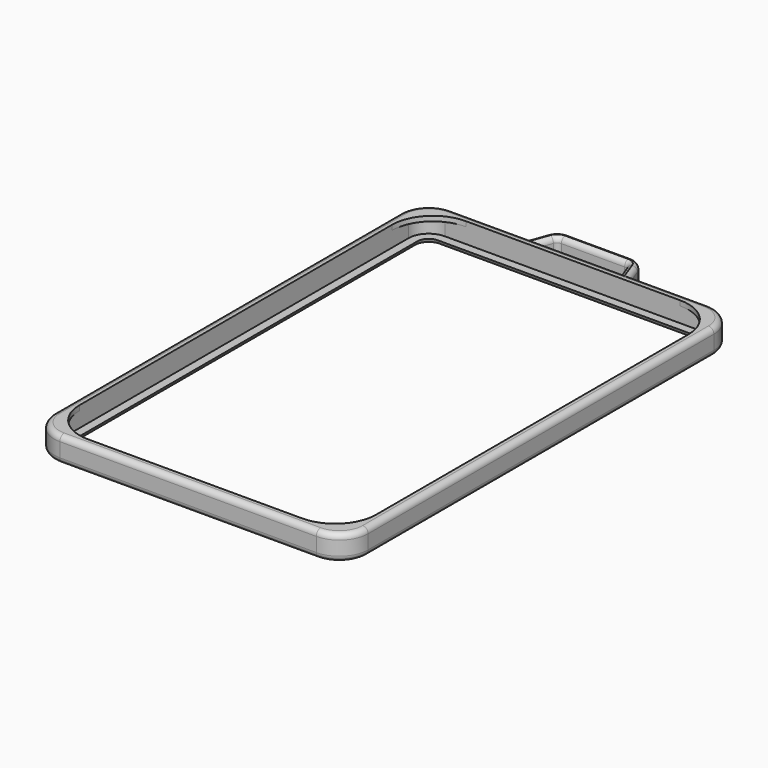
from build123d import *

# Parameters (mm, degrees)
F1_DEPTH      = 2.8
F3_DEPTH      = 0.9
F5_DEPTH      = 0.9
F7_DEPTH      = 3.7
F7_DEPTH_BACK = 0.9
F8_T1_DEPTH   = 79.2801919127
F8_T3_DEPTH   = 11.5995849236
F8_T5_DEPTH   = 47.0301919127
F8_T10_DEPTH  = 4.9923257792
F8_T15_DEPTH  = 20.1838214056
F8_T20_DEPTH  = 20.1838214056
F8_T26_DEPTH  = 20.1838214056
F8_T31_DEPTH  = 20.1838214056
F8_T36_DEPTH  = 20.1838214056
F8_T42_DEPTH  = 20.1838214056
F8_T45_ANGLE  = 90
F8_T47_ANGLE  = 90
F8_T49_ANGLE  = 90
F8_T51_ANGLE  = 90
F8_T53_ANGLE  = 90
F8_T57_DEPTH  = 16.7205008176
F8_T62_DEPTH  = 16.7205008176
F8_T67_DEPTH  = 16.7205008176
F8_T72_DEPTH  = 16.7205008176
F8_T75_ANGLE  = 90
F8_T77_ANGLE  = 90
F8_T81_DEPTH  = 16.7205008176
F8_T86_DEPTH  = 16.7205008176
F8_T91_DEPTH  = 16.7205008176
F8_T96_DEPTH  = 16.7205008176
F8_T99_ANGLE  = 90
F8_T101_ANGLE = 90
F8_T103_ANGLE = 90
F8_T105_ANGLE = 90
F8_T107_ANGLE = 90
F8_T109_ANGLE = 70
F8_T111_ANGLE = 70
F8_T115_DEPTH = 4.9923257792
F8_T120_DEPTH = 4.9923257792
F8_T123_ANGLE = 70
F8_T125_ANGLE = 70
F8_T129_DEPTH = 5.574678154
F8_T134_DEPTH = 5.574678154
F8_T137_ANGLE = 70
F8_T139_ANGLE = 70
F8_T143_DEPTH = 5.574678154
F8_T148_DEPTH = 5.574678154
F8_T151_ANGLE = 70
F8_T153_ANGLE = 70
F8_T157_DEPTH = 4.9923257792
F8_T163_DEPTH = 20.1838214056
F8_T168_DEPTH = 4.9923257792
F8_T175_DEPTH = 20.1838214056
F8_T180_DEPTH = 4.9923257792
F8_T187_DEPTH = 20.1838214056
F8_T192_DEPTH = 4.9923257792
F8_T199_DEPTH = 20.1838214056
F8_T204_DEPTH = 4.9923257792
F8_T211_DEPTH = 16.7205008176
F8_T216_DEPTH = 5.574678154
F8_T223_DEPTH = 5.574678154
F8_T227_DEPTH = 16.7205008176
F8_T235_DEPTH = 16.7205008176
F8_T240_DEPTH = 5.574678154
F8_T247_DEPTH = 5.574678154
F8_T251_DEPTH = 16.7205008176


# Not quite as in the source:
# - a fillet or chamfer that OpenCascade refuses, or shapes differently, is made with other operations: its cross-section is extruded or revolved along the edge and cut away or added


with BuildPart() as f1:
    # F0 (on Top) → F1 (new body)
    with BuildSketch(Plane.XY):
        with BuildLine():
            Line((-28.8, 39.6400959564), (-28.8, -39.6400959564))
            ThreePointArc((-28.8, -39.6400959564), (-27.2520874435, -43.3770874435), (-23.5150959564, -44.925))
            Line((-23.5150959564, -44.925), (23.5150959564, -44.925))
            ThreePointArc((23.5150959564, -44.925), (27.2520874435, -43.3770874435), (28.8, -39.6400959564))
            Line((28.8, -39.6400959564), (28.8, 39.6400959564))
            ThreePointArc((28.8, 39.6400959564), (27.2520874435, 43.3770874435), (23.5150959564, 44.925))
            Line((23.5150959564, 44.925), (-23.5150959564, 44.925))
            ThreePointArc((-23.5150959564, 44.925), (-27.2520874435, 43.3770874435), (-28.8, 39.6400959564))
        make_face()
        with BuildLine():
            ThreePointArc((-23.5150959564, -43.325), (-26.1207165936, -42.2457165936), (-27.2, -39.6400959564))
            Line((-27.2, -39.6400959564), (-27.2, 39.6400959564))
            ThreePointArc((-27.2, 39.6400959564), (-26.1207165936, 42.2457165936), (-23.5150959564, 43.325))
            Line((-23.5150959564, 43.325), (23.5150959564, 43.325))
            ThreePointArc((23.5150959564, 43.325), (26.1207165936, 42.2457165936), (27.2, 39.6400959564))
            Line((27.2, 39.6400959564), (27.2, -39.6400959564))
            ThreePointArc((27.2, -39.6400959564), (26.1207165936, -42.2457165936), (23.5150959564, -43.325))
            Line((23.5150959564, -43.325), (-23.5150959564, -43.325))
        make_face(mode=Mode.SUBTRACT)
    extrude(amount=F1_DEPTH)

    # F2 (on face) → F3 (join)
    with BuildSketch(Plane(origin=(0, 0, 0), x_dir=(1, 0, 0), z_dir=(0, 0, -1))):
        with BuildLine():
            Line((28.8, -39.6400959564), (28.8, 39.6400959564))
            ThreePointArc((28.8, 39.6400959564), (27.2520874435, 43.3770874435), (23.5150959564, 44.925))
            Line((23.5150959564, 44.925), (-23.5150959564, 44.925))
            ThreePointArc((-23.5150959564, 44.925), (-27.2520874435, 43.3770874435), (-28.8, 39.6400959564))
            Line((-28.8, 39.6400959564), (-28.8, -39.6400959564))
            ThreePointArc((-28.8, -39.6400959564), (-27.2520874435, -43.3770874435), (-23.5150959564, -44.925))
            Line((-23.5150959564, -44.925), (23.5150959564, -44.925))
            ThreePointArc((23.5150959564, -44.925), (27.2520874435, -43.3770874435), (28.8, -39.6400959564))
        make_face()
        with BuildLine():
            Line((-27.2, -39.6400959564), (-27.2, 39.6400959564))
            ThreePointArc((-27.2, 39.6400959564), (-26.1207165936, 42.2457165936), (-23.5150959564, 43.325))
            Line((-23.5150959564, 43.325), (23.5150959564, 43.325))
            ThreePointArc((23.5150959564, 43.325), (26.1207165936, 42.2457165936), (27.2, 39.6400959564))
            Line((27.2, 39.6400959564), (27.2, -39.6400959564))
            ThreePointArc((27.2, -39.6400959564), (26.1207165936, -42.2457165936), (23.5150959564, -43.325))
            Line((23.5150959564, -43.325), (-23.5150959564, -43.325))
            ThreePointArc((-23.5150959564, -43.325), (-26.1207165936, -42.2457165936), (-27.2, -39.6400959564))
        make_face(mode=Mode.SUBTRACT)
        with BuildLine():
            ThreePointArc((-23.5150959564, 43.325), (-26.1207165936, 42.2457165936), (-27.2, 39.6400959564))
            Line((-27.2, 39.6400959564), (-27.2, -39.6400959564))
            ThreePointArc((-27.2, -39.6400959564), (-26.1207165936, -42.2457165936), (-23.5150959564, -43.325))
            Line((-23.5150959564, -43.325), (23.5150959564, -43.325))
            ThreePointArc((23.5150959564, -43.325), (26.1207165936, -42.2457165936), (27.2, -39.6400959564))
            Line((27.2, -39.6400959564), (27.2, 39.6400959564))
            ThreePointArc((27.2, 39.6400959564), (26.1207165936, 42.2457165936), (23.5150959564, 43.325))
            Line((23.5150959564, 43.325), (-23.5150959564, 43.325))
        make_face()
        with BuildLine():
            Line((-25.6, -39.6400959564), (-25.6, 39.6400959564))
            ThreePointArc((-25.6, 39.6400959564), (-24.9893457437, 41.1143457437), (-23.5150959564, 41.725))
            Line((-23.5150959564, 41.725), (23.5150959564, 41.725))
            ThreePointArc((23.5150959564, 41.725), (24.9893457437, 41.1143457437), (25.6, 39.6400959564))
            Line((25.6, 39.6400959564), (25.6, -39.6400959564))
            ThreePointArc((25.6, -39.6400959564), (24.9893457437, -41.1143457437), (23.5150959564, -41.725))
            Line((23.5150959564, -41.725), (-23.5150959564, -41.725))
            ThreePointArc((-23.5150959564, -41.725), (-24.9893457437, -41.1143457437), (-25.6, -39.6400959564))
        make_face(mode=Mode.SUBTRACT)
    extrude(amount=F3_DEPTH)

    # F4 (on face) → F5 (join)
    with BuildSketch(Plane.XY.offset(2.8)):
        with BuildLine():
            Line((-23.5150959564, -44.925), (23.5150959564, -44.925))
            ThreePointArc((23.5150959564, -44.925), (27.2520874435, -43.3770874435), (28.8, -39.6400959564))
            Line((28.8, -39.6400959564), (28.8, 39.6400959564))
            ThreePointArc((28.8, 39.6400959564), (27.2520874435, 43.3770874435), (23.5150959564, 44.925))
            Line((23.5150959564, 44.925), (-23.5150959564, 44.925))
            ThreePointArc((-23.5150959564, 44.925), (-27.2520874435, 43.3770874435), (-28.8, 39.6400959564))
            Line((-28.8, 39.6400959564), (-28.8, -39.6400959564))
            ThreePointArc((-28.8, -39.6400959564), (-27.2520874435, -43.3770874435), (-23.5150959564, -44.925))
        make_face()
        with BuildLine():
            Line((19.6523542566, 43.325), (23.5150959564, 43.325))
            ThreePointArc((23.5150959564, 43.325), (26.1207165936, 42.2457165936), (27.2, 39.6400959564))
            Line((27.2, 39.6400959564), (27.2, 35.7773542566))
            Line((27.2, 35.7773542566), (27.2, -35.7773542566))
            Line((27.2, -35.7773542566), (27.2, -39.6400959564))
            ThreePointArc((27.2, -39.6400959564), (26.1207165936, -42.2457165936), (23.5150959564, -43.325))
            Line((23.5150959564, -43.325), (19.6523542566, -43.325))
            Line((19.6523542566, -43.325), (-19.6523542566, -43.325))
            Line((-19.6523542566, -43.325), (-23.5150959564, -43.325))
            ThreePointArc((-23.5150959564, -43.325), (-26.1207165936, -42.2457165936), (-27.2, -39.6400959564))
            Line((-27.2, -39.6400959564), (-27.2, -35.7773542566))
            Line((-27.2, -35.7773542566), (-27.2, 35.7773542566))
            Line((-27.2, 35.7773542566), (-27.2, 39.6400959564))
            ThreePointArc((-27.2, 39.6400959564), (-26.1207165936, 42.2457165936), (-23.5150959564, 43.325))
            Line((-23.5150959564, 43.325), (-19.6523542566, 43.325))
            Line((-19.6523542566, 43.325), (19.6523542566, 43.325))
        make_face(mode=Mode.SUBTRACT)
        with BuildLine():
            ThreePointArc((-27.2, 35.7773542566), (-24.9893457437, 41.1143457437), (-19.6523542566, 43.325))
            Line((-19.6523542566, 43.325), (-23.5150959564, 43.325))
            ThreePointArc((-23.5150959564, 43.325), (-26.1207165936, 42.2457165936), (-27.2, 39.6400959564))
            Line((-27.2, 39.6400959564), (-27.2, 35.7773542566))
        make_face()
        with BuildLine():
            ThreePointArc((27.2, 39.6400959564), (26.1207165936, 42.2457165936), (23.5150959564, 43.325))
            Line((23.5150959564, 43.325), (19.6523542566, 43.325))
            ThreePointArc((19.6523542566, 43.325), (24.9893457437, 41.1143457437), (27.2, 35.7773542566))
            Line((27.2, 35.7773542566), (27.2, 39.6400959564))
        make_face()
        with BuildLine():
            Line((27.2, -39.6400959564), (27.2, -35.7773542566))
            ThreePointArc((27.2, -35.7773542566), (24.9893457437, -41.1143457437), (19.6523542566, -43.325))
            Line((19.6523542566, -43.325), (23.5150959564, -43.325))
            ThreePointArc((23.5150959564, -43.325), (26.1207165936, -42.2457165936), (27.2, -39.6400959564))
        make_face()
        with BuildLine():
            ThreePointArc((-19.6523542566, -43.325), (-24.9893457437, -41.1143457437), (-27.2, -35.7773542566))
            Line((-27.2, -35.7773542566), (-27.2, -39.6400959564))
            ThreePointArc((-27.2, -39.6400959564), (-26.1207165936, -42.2457165936), (-23.5150959564, -43.325))
            Line((-23.5150959564, -43.325), (-19.6523542566, -43.325))
        make_face()
    extrude(amount=F5_DEPTH)

    # F6 (on Top) → F7 (join, two sides)
    with BuildSketch(Plane.XY) as f7_sk:
        with BuildLine():
            Line((-9.2945951388, 44.925), (-7.5919107028, 44.925))
            Line((-7.5919107028, 44.925), (-6.7394850826, 47.2670201433))
            ThreePointArc((-6.7394850826, 47.2670201433), (-6.3733688981, 47.7441520443), (-5.7997924618, 47.925))
            Line((-5.7997924618, 47.925), (5.7997924618, 47.925))
            ThreePointArc((5.7997924618, 47.925), (6.3733688981, 47.7441520443), (6.7394850826, 47.2670201433))
            Line((6.7394850826, 47.2670201433), (7.5919107028, 44.925))
            Line((7.5919107028, 44.925), (9.2945951388, 44.925))
            Line((9.2945951388, 44.925), (8.2429932758, 47.8142523726))
            ThreePointArc((8.2429932758, 47.8142523726), (7.2910911963, 49.0547953152), (5.7997924618, 49.525))
            Line((5.7997924618, 49.525), (-5.7997924618, 49.525))
            ThreePointArc((-5.7997924618, 49.525), (-7.2910911963, 49.0547953152), (-8.2429932758, 47.8142523726))
            Line((-8.2429932758, 47.8142523726), (-9.2945951388, 44.925))
        make_face()
    extrude(amount=F7_DEPTH)
    extrude(f7_sk.sketch, amount=-F7_DEPTH_BACK)

    # F8: fillet of radius 1 on 25 edges, made by hand

    # F8_s2 → F8_t1 (cut)
    with BuildSketch(Plane.XZ.offset(-39.6400959564)):
        with BuildLine():
            ThreePointArc((-28.8, 2.7), (-28.5071067812, 3.4071067812), (-27.8, 3.7))
            Line((-27.8, 3.7), (-27.8, 3.72))
            Line((-27.8, 3.72), (-28.82, 3.72))
            Line((-28.82, 3.72), (-28.82, 2.7))
            Line((-28.82, 2.7), (-28.8, 2.7))
        make_face()
        with BuildLine():
            ThreePointArc((-28.8, 0.1), (-28.5071067812, -0.6071067812), (-27.8, -0.9))
            Line((-27.8, -0.9), (-27.8, -0.92))
            Line((-27.8, -0.92), (-28.82, -0.92))
            Line((-28.82, -0.92), (-28.82, 0.1))
            Line((-28.82, 0.1), (-28.8, 0.1))
        make_face()
        with BuildLine():
            ThreePointArc((-26.5949874371, -0.9), (-25.9241670439, -0.6416198487), (-25.6, 0))
            Line((-25.6, 0), (-25.5801002513, -0.002))
            ThreePointArc((-25.5801002513, -0.002), (-25.58, -0.45), (-25.58, -0.9))
            Line((-25.58, -0.9), (-25.6, -0.92))
            Line((-25.6, -0.92), (-26.5949874371, -0.92))
            Line((-26.5949874371, -0.92), (-26.5949874371, -0.9))
        make_face()
        with BuildLine():
            ThreePointArc((27.8, 3.7), (28.5071067812, 3.4071067812), (28.8, 2.7))
            Line((28.8, 2.7), (28.82, 2.7))
            Line((28.82, 2.7), (28.82, 3.72))
            Line((28.82, 3.72), (27.8, 3.72))
            Line((27.8, 3.72), (27.8, 3.7))
        make_face()
        with BuildLine():
            ThreePointArc((27.8, -0.9), (28.5071067812, -0.6071067812), (28.8, 0.1))
            Line((28.8, 0.1), (28.82, 0.1))
            Line((28.82, 0.1), (28.82, -0.92))
            Line((28.82, -0.92), (27.8, -0.92))
            Line((27.8, -0.92), (27.8, -0.9))
        make_face()
        with BuildLine():
            ThreePointArc((26.5949874371, -0.9), (25.9241670439, -0.6416198487), (25.6, 0))
            Line((25.6, 0), (25.5801002513, -0.002))
            ThreePointArc((25.5801002513, -0.002), (25.58, -0.45), (25.58, -0.9))
            Line((25.58, -0.9), (25.6, -0.92))
            Line((25.6, -0.92), (26.5949874371, -0.92))
            Line((26.5949874371, -0.92), (26.5949874371, -0.9))
        make_face()
    extrude(amount=F8_T1_DEPTH, mode=Mode.SUBTRACT)

    # F8_s4 → F8_t3 (cut)
    with BuildSketch(Plane.YZ.offset(-5.7997924618)):
        with BuildLine():
            ThreePointArc((48.525, -0.9), (49.2321067812, -0.6071067812), (49.525, 0.1))
            Line((49.525, 0.1), (49.545, 0.1))
            Line((49.545, 0.1), (49.545, -0.92))
            Line((49.545, -0.92), (48.525, -0.92))
            Line((48.525, -0.92), (48.525, -0.9))
        make_face()
        with BuildLine():
            ThreePointArc((48.525, 3.7), (49.2321067812, 3.4071067812), (49.525, 2.7))
            Line((49.525, 2.7), (49.545, 2.7))
            Line((49.545, 2.7), (49.545, 3.72))
            Line((49.545, 3.72), (48.525, 3.72))
            Line((48.525, 3.72), (48.525, 3.7))
        make_face()
        with BuildLine():
            ThreePointArc((48.925, -0.9), (48.2178932188, -0.6071067812), (47.925, 0.1))
            Line((47.925, 0.1), (47.905, 0.1))
            Line((47.905, 0.1), (47.905, -0.92))
            Line((47.905, -0.92), (48.925, -0.92))
            Line((48.925, -0.92), (48.925, -0.9))
        make_face()
        with BuildLine():
            ThreePointArc((48.925, 3.7), (48.2178932188, 3.4071067812), (47.925, 2.7))
            Line((47.925, 2.7), (47.905, 2.7))
            Line((47.905, 2.7), (47.905, 3.72))
            Line((47.905, 3.72), (48.925, 3.72))
            Line((48.925, 3.72), (48.925, 3.7))
        make_face()
    extrude(amount=F8_T3_DEPTH, mode=Mode.SUBTRACT)

    # F8_s6 → F8_t5 (cut)
    with BuildSketch(Plane.YZ.offset(-23.5150959564)):
        with BuildLine():
            ThreePointArc((-43.925, 3.7), (-44.6321067812, 3.4071067812), (-44.925, 2.7))
            Line((-44.925, 2.7), (-44.945, 2.7))
            Line((-44.945, 2.7), (-44.945, 3.72))
            Line((-44.945, 3.72), (-43.925, 3.72))
            Line((-43.925, 3.72), (-43.925, 3.7))
        make_face()
        with BuildLine():
            ThreePointArc((-43.925, -0.9), (-44.6321067812, -0.6071067812), (-44.925, 0.1))
            Line((-44.925, 0.1), (-44.945, 0.1))
            Line((-44.945, 0.1), (-44.945, -0.92))
            Line((-44.945, -0.92), (-43.925, -0.92))
            Line((-43.925, -0.92), (-43.925, -0.9))
        make_face()
        with BuildLine():
            ThreePointArc((-42.7199874371, -0.9), (-42.0491670439, -0.6416198487), (-41.725, 0))
            Line((-41.725, 0), (-41.7051002513, -0.002))
            ThreePointArc((-41.7051002513, -0.002), (-41.705, -0.45), (-41.705, -0.9))
            Line((-41.705, -0.9), (-41.725, -0.92))
            Line((-41.725, -0.92), (-42.7199874371, -0.92))
            Line((-42.7199874371, -0.92), (-42.7199874371, -0.9))
        make_face()
        with BuildLine():
            ThreePointArc((42.7199874371, -0.9), (42.0491670439, -0.6416198487), (41.725, 0))
            Line((41.725, 0), (41.7051002513, -0.002))
            ThreePointArc((41.7051002513, -0.002), (41.705, -0.45), (41.705, -0.9))
            Line((41.705, -0.9), (41.725, -0.92))
            Line((41.725, -0.92), (42.7199874371, -0.92))
            Line((42.7199874371, -0.92), (42.7199874371, -0.9))
        make_face()
    extrude(amount=F8_T5_DEPTH, mode=Mode.SUBTRACT)


with BuildPart() as f8_tool8:
    # F8_s9 → F8_t10 (new body)
    with BuildSketch(Plane(origin=(12.6954814761, 34.8805486848, 0), x_dir=(0, 0, 1), z_dir=(0.3420201433, 0.9396926208, 0))):
        with BuildLine():
            ThreePointArc((3.7, -23.499317404), (3.4071067812, -22.7922106228), (2.7, -22.499317404))
            Line((2.7, -22.499317404), (2.7, -22.479317404))
            Line((2.7, -22.479317404), (3.72, -22.479317404))
            Line((3.72, -22.479317404), (3.72, -23.499317404))
            Line((3.72, -23.499317404), (3.7, -23.499317404))
        make_face()
    extrude(amount=F8_T10_DEPTH)

    split(bisect_by=Plane.XZ.offset(-44.925), keep=Keep.BOTTOM)


with BuildPart() as f1_1:
    add(f1.part)

    # F8_t7: cut F8_tool8
    add(f8_tool8.part, mode=Mode.SUBTRACT)


with BuildPart() as f8_tool13:
    # F8_s14 → F8_t15 (new body)
    with BuildSketch(Plane.YZ.offset(-10.0919107028)):
        with BuildLine():
            ThreePointArc((43.925, -0.9), (44.6321067812, -0.6071067812), (44.925, 0.1))
            Line((44.925, 0.1), (44.945, 0.1))
            Line((44.945, 0.1), (44.945, -0.92))
            Line((44.945, -0.92), (43.925, -0.92))
            Line((43.925, -0.92), (43.925, -0.9))
        make_face()
    extrude(amount=F8_T15_DEPTH)

    split(bisect_by=Plane(origin=(-22.6459507305, 8.2424519926, 0), x_dir=(0, 0, 1), z_dir=(-0.9396926208, 0.3420201433, 0)), keep=Keep.TOP)


with BuildPart() as f1_2:
    add(f1_1.part)

    # F8_t12: cut F8_tool13
    add(f8_tool13.part, mode=Mode.SUBTRACT)


with BuildPart() as f8_tool18:
    # F8_s19 → F8_t20 (new body)
    with BuildSketch(Plane.YZ.offset(-10.0919107028)):
        with BuildLine():
            ThreePointArc((43.925, -0.9), (44.6321067812, -0.6071067812), (44.925, 0.1))
            Line((44.925, 0.1), (44.945, 0.1))
            Line((44.945, 0.1), (44.945, -0.92))
            Line((44.945, -0.92), (43.925, -0.92))
            Line((43.925, -0.92), (43.925, -0.9))
        make_face()
    extrude(amount=F8_T20_DEPTH)

    split(bisect_by=Plane(origin=(21.1424425373, 7.6952197632, 0), x_dir=(0, 0, 1), z_dir=(-0.9396926208, -0.3420201433, 0)), keep=Keep.TOP)

    split(bisect_by=Plane(origin=(-21.1424425373, 7.6952197632, 0), x_dir=(0, 0, 1), z_dir=(0.9396926208, -0.3420201433, 0)), keep=Keep.TOP)


with BuildPart() as f1_3:
    add(f1_2.part)

    # F8_t17: cut F8_tool18
    add(f8_tool18.part, mode=Mode.SUBTRACT)


with BuildPart() as f8_tool24:
    # F8_s25 → F8_t26 (new body)
    with BuildSketch(Plane.YZ.offset(-10.0919107028)):
        with BuildLine():
            ThreePointArc((43.925, -0.9), (44.6321067812, -0.6071067812), (44.925, 0.1))
            Line((44.925, 0.1), (44.945, 0.1))
            Line((44.945, 0.1), (44.945, -0.92))
            Line((44.945, -0.92), (43.925, -0.92))
            Line((43.925, -0.92), (43.925, -0.9))
        make_face()
    extrude(amount=F8_T26_DEPTH)

    split(bisect_by=Plane(origin=(22.6459507305, 8.2424519926, 0), x_dir=(0, 0, 1), z_dir=(0.9396926208, 0.3420201433, 0)), keep=Keep.TOP)


with BuildPart() as f1_4:
    add(f1_3.part)

    # F8_t23: cut F8_tool24
    add(f8_tool24.part, mode=Mode.SUBTRACT)


with BuildPart() as f8_tool29:
    # F8_s30 → F8_t31 (new body)
    with BuildSketch(Plane.YZ.offset(10.0919107028)):
        with BuildLine():
            ThreePointArc((43.925, 3.7), (44.6321067812, 3.4071067812), (44.925, 2.7))
            Line((44.925, 2.7), (44.945, 2.7))
            Line((44.945, 2.7), (44.945, 3.72))
            Line((44.945, 3.72), (43.925, 3.72))
            Line((43.925, 3.72), (43.925, 3.7))
        make_face()
    extrude(amount=-F8_T31_DEPTH)

    split(bisect_by=Plane(origin=(22.6459507305, 8.2424519926, 0), x_dir=(0, 0, 1), z_dir=(0.9396926208, 0.3420201433, 0)), keep=Keep.TOP)


with BuildPart() as f1_5:
    add(f1_4.part)

    # F8_t28: cut F8_tool29
    add(f8_tool29.part, mode=Mode.SUBTRACT)


with BuildPart() as f8_tool34:
    # F8_s35 → F8_t36 (new body)
    with BuildSketch(Plane.YZ.offset(10.0919107028)):
        with BuildLine():
            ThreePointArc((43.925, 3.7), (44.6321067812, 3.4071067812), (44.925, 2.7))
            Line((44.925, 2.7), (44.945, 2.7))
            Line((44.945, 2.7), (44.945, 3.72))
            Line((44.945, 3.72), (43.925, 3.72))
            Line((43.925, 3.72), (43.925, 3.7))
        make_face()
    extrude(amount=-F8_T36_DEPTH)

    split(bisect_by=Plane(origin=(21.1424425373, 7.6952197632, 0), x_dir=(0, 0, 1), z_dir=(-0.9396926208, -0.3420201433, 0)), keep=Keep.TOP)

    split(bisect_by=Plane(origin=(-21.1424425373, 7.6952197632, 0), x_dir=(0, 0, 1), z_dir=(0.9396926208, -0.3420201433, 0)), keep=Keep.TOP)


with BuildPart() as f1_6:
    add(f1_5.part)

    # F8_t33: cut F8_tool34
    add(f8_tool34.part, mode=Mode.SUBTRACT)


with BuildPart() as f8_tool40:
    # F8_s41 → F8_t42 (new body)
    with BuildSketch(Plane.YZ.offset(10.0919107028)):
        with BuildLine():
            ThreePointArc((43.925, 3.7), (44.6321067812, 3.4071067812), (44.925, 2.7))
            Line((44.925, 2.7), (44.945, 2.7))
            Line((44.945, 2.7), (44.945, 3.72))
            Line((44.945, 3.72), (43.925, 3.72))
            Line((43.925, 3.72), (43.925, 3.7))
        make_face()
    extrude(amount=-F8_T42_DEPTH)

    split(bisect_by=Plane(origin=(-22.6459507305, 8.2424519926, 0), x_dir=(0, 0, 1), z_dir=(-0.9396926208, 0.3420201433, 0)), keep=Keep.TOP)


with BuildPart() as f1_7:
    add(f1_6.part)

    # F8_t39: cut F8_tool40
    add(f8_tool40.part, mode=Mode.SUBTRACT)

    # F8_s44 → F8_t45 (revolve, cut)
    with BuildSketch(Plane.YZ.offset(-23.5150959564)):
        with BuildLine():
            ThreePointArc((44.925, 2.7), (44.6321067812, 3.4071067812), (43.925, 3.7))
            Line((43.925, 3.7), (43.925, 3.72))
            Line((43.925, 3.72), (44.945, 3.72))
            Line((44.945, 3.72), (44.945, 2.7))
            Line((44.945, 2.7), (44.925, 2.7))
        make_face()
    revolve(axis=Axis((-23.5150959564, 39.6400959564, 3.7), (0, 0, 1)), revolution_arc=F8_T45_ANGLE, mode=Mode.SUBTRACT)

    # F8_s46 → F8_t47 (revolve, cut)
    with BuildSketch(Plane.XZ.offset(-39.6400959564)):
        with BuildLine():
            ThreePointArc((-28.8, 0.1), (-28.5071067812, -0.6071067812), (-27.8, -0.9))
            Line((-27.8, -0.9), (-27.8, -0.92))
            Line((-27.8, -0.92), (-28.82, -0.92))
            Line((-28.82, -0.92), (-28.82, 0.1))
            Line((-28.82, 0.1), (-28.8, 0.1))
        make_face()
    revolve(axis=Axis((-23.5150959564, 39.6400959564, -0.9), (0, 0, -1)), revolution_arc=F8_T47_ANGLE, mode=Mode.SUBTRACT)

    # F8_s48 → F8_t49 (revolve, cut)
    with BuildSketch(Plane.XZ.offset(39.6400959564)):
        with BuildLine():
            ThreePointArc((-27.8, 3.7), (-28.5071067812, 3.4071067812), (-28.8, 2.7))
            Line((-28.8, 2.7), (-28.82, 2.7))
            Line((-28.82, 2.7), (-28.82, 3.72))
            Line((-28.82, 3.72), (-27.8, 3.72))
            Line((-27.8, 3.72), (-27.8, 3.7))
        make_face()
    revolve(axis=Axis((-23.5150959564, -39.6400959564, 3.7), (0, 0, 1)), revolution_arc=F8_T49_ANGLE, mode=Mode.SUBTRACT)

    # F8_s50 → F8_t51 (revolve, cut)
    with BuildSketch(Plane.YZ.offset(23.5150959564)):
        with BuildLine():
            ThreePointArc((-43.925, 3.7), (-44.6321067812, 3.4071067812), (-44.925, 2.7))
            Line((-44.925, 2.7), (-44.945, 2.7))
            Line((-44.945, 2.7), (-44.945, 3.72))
            Line((-44.945, 3.72), (-43.925, 3.72))
            Line((-43.925, 3.72), (-43.925, 3.7))
        make_face()
    revolve(axis=Axis((23.5150959564, -39.6400959564, 3.7), (0, 0, 1)), revolution_arc=F8_T51_ANGLE, mode=Mode.SUBTRACT)

    # F8_s52 → F8_t53 (revolve, cut)
    with BuildSketch(Plane.XZ.offset(-39.6400959564)):
        with BuildLine():
            ThreePointArc((27.8, 3.7), (28.5071067812, 3.4071067812), (28.8, 2.7))
            Line((28.8, 2.7), (28.82, 2.7))
            Line((28.82, 2.7), (28.82, 3.72))
            Line((28.82, 3.72), (27.8, 3.72))
            Line((27.8, 3.72), (27.8, 3.7))
        make_face()
    revolve(axis=Axis((23.5150959564, 39.6400959564, 3.7), (0, 0, 1)), revolution_arc=F8_T53_ANGLE, mode=Mode.SUBTRACT)


with BuildPart() as f8_tool55:
    # F8_s56 → F8_t57 (new body)
    with BuildSketch(Plane.YZ.offset(23.5150959564)):
        with BuildLine():
            ThreePointArc((43.925, 3.7), (44.6321067812, 3.4071067812), (44.925, 2.7))
            Line((44.925, 2.7), (44.945, 2.7))
            Line((44.945, 2.7), (44.945, 3.72))
            Line((44.945, 3.72), (43.925, 3.72))
            Line((43.925, 3.72), (43.925, 3.7))
        make_face()
    extrude(amount=-F8_T57_DEPTH)

    split(bisect_by=Plane(origin=(22.6459507305, 8.2424519926, 0), x_dir=(0, 0, 1), z_dir=(0.9396926208, 0.3420201433, 0)), keep=Keep.TOP)


with BuildPart() as f1_8:
    add(f1_7.part)

    # F8_t54: cut F8_tool55
    add(f8_tool55.part, mode=Mode.SUBTRACT)


with BuildPart() as f8_tool60:
    # F8_s61 → F8_t62 (new body)
    with BuildSketch(Plane.YZ.offset(23.5150959564)):
        with BuildLine():
            ThreePointArc((43.925, 3.7), (44.6321067812, 3.4071067812), (44.925, 2.7))
            Line((44.925, 2.7), (44.945, 2.7))
            Line((44.945, 2.7), (44.945, 3.72))
            Line((44.945, 3.72), (43.925, 3.72))
            Line((43.925, 3.72), (43.925, 3.7))
        make_face()
    extrude(amount=-F8_T62_DEPTH)

    split(bisect_by=Plane(origin=(21.1424425373, 7.6952197632, 0), x_dir=(0, 0, 1), z_dir=(-0.9396926208, -0.3420201433, 0)), keep=Keep.TOP)


with BuildPart() as f1_9:
    add(f1_8.part)

    # F8_t59: cut F8_tool60
    add(f8_tool60.part, mode=Mode.SUBTRACT)


with BuildPart() as f8_tool65:
    # F8_s66 → F8_t67 (new body)
    with BuildSketch(Plane.YZ.offset(-6.7945951388)):
        with BuildLine():
            ThreePointArc((43.925, 3.7), (44.6321067812, 3.4071067812), (44.925, 2.7))
            Line((44.925, 2.7), (44.945, 2.7))
            Line((44.945, 2.7), (44.945, 3.72))
            Line((44.945, 3.72), (43.925, 3.72))
            Line((43.925, 3.72), (43.925, 3.7))
        make_face()
    extrude(amount=-F8_T67_DEPTH)

    split(bisect_by=Plane(origin=(-21.1424425373, 7.6952197632, 0), x_dir=(0, 0, 1), z_dir=(0.9396926208, -0.3420201433, 0)), keep=Keep.TOP)


with BuildPart() as f1_10:
    add(f1_9.part)

    # F8_t64: cut F8_tool65
    add(f8_tool65.part, mode=Mode.SUBTRACT)


with BuildPart() as f8_tool70:
    # F8_s71 → F8_t72 (new body)
    with BuildSketch(Plane.YZ.offset(-6.7945951388)):
        with BuildLine():
            ThreePointArc((43.925, 3.7), (44.6321067812, 3.4071067812), (44.925, 2.7))
            Line((44.925, 2.7), (44.945, 2.7))
            Line((44.945, 2.7), (44.945, 3.72))
            Line((44.945, 3.72), (43.925, 3.72))
            Line((43.925, 3.72), (43.925, 3.7))
        make_face()
    extrude(amount=-F8_T72_DEPTH)

    split(bisect_by=Plane(origin=(-22.6459507305, 8.2424519926, 0), x_dir=(0, 0, 1), z_dir=(-0.9396926208, 0.3420201433, 0)), keep=Keep.TOP)


with BuildPart() as f1_11:
    add(f1_10.part)

    # F8_t69: cut F8_tool70
    add(f8_tool70.part, mode=Mode.SUBTRACT)

    # F8_s74 → F8_t75 (revolve, cut)
    with BuildSketch(Plane.YZ.offset(-23.5150959564)):
        with BuildLine():
            ThreePointArc((-44.925, 0.1), (-44.6321067812, -0.6071067812), (-43.925, -0.9))
            Line((-43.925, -0.9), (-43.925, -0.92))
            Line((-43.925, -0.92), (-44.945, -0.92))
            Line((-44.945, -0.92), (-44.945, 0.1))
            Line((-44.945, 0.1), (-44.925, 0.1))
        make_face()
    revolve(axis=Axis((-23.5150959564, -39.6400959564, -0.9), (0, 0, -1)), revolution_arc=F8_T75_ANGLE, mode=Mode.SUBTRACT)

    # F8_s76 → F8_t77 (revolve, cut)
    with BuildSketch(Plane.XZ.offset(39.6400959564)):
        with BuildLine():
            ThreePointArc((27.8, -0.9), (28.5071067812, -0.6071067812), (28.8, 0.1))
            Line((28.8, 0.1), (28.82, 0.1))
            Line((28.82, 0.1), (28.82, -0.92))
            Line((28.82, -0.92), (27.8, -0.92))
            Line((27.8, -0.92), (27.8, -0.9))
        make_face()
    revolve(axis=Axis((23.5150959564, -39.6400959564, -0.9), (0, 0, -1)), revolution_arc=F8_T77_ANGLE, mode=Mode.SUBTRACT)


with BuildPart() as f8_tool79:
    # F8_s80 → F8_t81 (new body)
    with BuildSketch(Plane.YZ.offset(-23.5150959564)):
        with BuildLine():
            ThreePointArc((43.925, -0.9), (44.6321067812, -0.6071067812), (44.925, 0.1))
            Line((44.925, 0.1), (44.945, 0.1))
            Line((44.945, 0.1), (44.945, -0.92))
            Line((44.945, -0.92), (43.925, -0.92))
            Line((43.925, -0.92), (43.925, -0.9))
        make_face()
    extrude(amount=F8_T81_DEPTH)

    split(bisect_by=Plane(origin=(-22.6459507305, 8.2424519926, 0), x_dir=(0, 0, 1), z_dir=(-0.9396926208, 0.3420201433, 0)), keep=Keep.TOP)


with BuildPart() as f1_12:
    add(f1_11.part)

    # F8_t78: cut F8_tool79
    add(f8_tool79.part, mode=Mode.SUBTRACT)


with BuildPart() as f8_tool84:
    # F8_s85 → F8_t86 (new body)
    with BuildSketch(Plane.YZ.offset(-23.5150959564)):
        with BuildLine():
            ThreePointArc((43.925, -0.9), (44.6321067812, -0.6071067812), (44.925, 0.1))
            Line((44.925, 0.1), (44.945, 0.1))
            Line((44.945, 0.1), (44.945, -0.92))
            Line((44.945, -0.92), (43.925, -0.92))
            Line((43.925, -0.92), (43.925, -0.9))
        make_face()
    extrude(amount=F8_T86_DEPTH)

    split(bisect_by=Plane(origin=(-21.1424425373, 7.6952197632, 0), x_dir=(0, 0, 1), z_dir=(0.9396926208, -0.3420201433, 0)), keep=Keep.TOP)


with BuildPart() as f1_13:
    add(f1_12.part)

    # F8_t83: cut F8_tool84
    add(f8_tool84.part, mode=Mode.SUBTRACT)


with BuildPart() as f8_tool89:
    # F8_s90 → F8_t91 (new body)
    with BuildSketch(Plane.YZ.offset(6.7945951388)):
        with BuildLine():
            ThreePointArc((43.925, -0.9), (44.6321067812, -0.6071067812), (44.925, 0.1))
            Line((44.925, 0.1), (44.945, 0.1))
            Line((44.945, 0.1), (44.945, -0.92))
            Line((44.945, -0.92), (43.925, -0.92))
            Line((43.925, -0.92), (43.925, -0.9))
        make_face()
    extrude(amount=F8_T91_DEPTH)

    split(bisect_by=Plane(origin=(21.1424425373, 7.6952197632, 0), x_dir=(0, 0, 1), z_dir=(-0.9396926208, -0.3420201433, 0)), keep=Keep.TOP)


with BuildPart() as f1_14:
    add(f1_13.part)

    # F8_t88: cut F8_tool89
    add(f8_tool89.part, mode=Mode.SUBTRACT)


with BuildPart() as f8_tool94:
    # F8_s95 → F8_t96 (new body)
    with BuildSketch(Plane.YZ.offset(6.7945951388)):
        with BuildLine():
            ThreePointArc((43.925, -0.9), (44.6321067812, -0.6071067812), (44.925, 0.1))
            Line((44.925, 0.1), (44.945, 0.1))
            Line((44.945, 0.1), (44.945, -0.92))
            Line((44.945, -0.92), (43.925, -0.92))
            Line((43.925, -0.92), (43.925, -0.9))
        make_face()
    extrude(amount=F8_T96_DEPTH)

    split(bisect_by=Plane(origin=(22.6459507305, 8.2424519926, 0), x_dir=(0, 0, 1), z_dir=(0.9396926208, 0.3420201433, 0)), keep=Keep.TOP)


with BuildPart() as f1_15:
    add(f1_14.part)

    # F8_t93: cut F8_tool94
    add(f8_tool94.part, mode=Mode.SUBTRACT)

    # F8_s98 → F8_t99 (revolve, cut)
    with BuildSketch(Plane.YZ.offset(23.5150959564)):
        with BuildLine():
            ThreePointArc((43.925, -0.9), (44.6321067812, -0.6071067812), (44.925, 0.1))
            Line((44.925, 0.1), (44.945, 0.1))
            Line((44.945, 0.1), (44.945, -0.92))
            Line((44.945, -0.92), (43.925, -0.92))
            Line((43.925, -0.92), (43.925, -0.9))
        make_face()
    revolve(axis=Axis((23.5150959564, 39.6400959564, -0.9), (0, 0, -1)), revolution_arc=F8_T99_ANGLE, mode=Mode.SUBTRACT)

    # F8_s100 → F8_t101 (revolve, cut)
    with BuildSketch(Plane.YZ.offset(-23.5150959564)):
        with BuildLine():
            ThreePointArc((42.7199874371, -0.9), (42.0491670439, -0.6416198487), (41.725, 0))
            Line((41.725, 0), (41.7051002513, -0.002))
            ThreePointArc((41.7051002513, -0.002), (41.705, -0.45), (41.705, -0.9))
            Line((41.705, -0.9), (41.725, -0.92))
            Line((41.725, -0.92), (42.7199874371, -0.92))
            Line((42.7199874371, -0.92), (42.7199874371, -0.9))
        make_face()
    revolve(axis=Axis((-23.5150959564, 39.6400959564, -0.9), (0, 0, 1)), revolution_arc=F8_T101_ANGLE, mode=Mode.SUBTRACT)

    # F8_s102 → F8_t103 (revolve, cut)
    with BuildSketch(Plane.XZ.offset(39.6400959564)):
        with BuildLine():
            ThreePointArc((-26.5949874371, -0.9), (-25.9241670439, -0.6416198487), (-25.6, 0))
            Line((-25.6, 0), (-25.5801002513, -0.002))
            ThreePointArc((-25.5801002513, -0.002), (-25.58, -0.45), (-25.58, -0.9))
            Line((-25.58, -0.9), (-25.6, -0.92))
            Line((-25.6, -0.92), (-26.5949874371, -0.92))
            Line((-26.5949874371, -0.92), (-26.5949874371, -0.9))
        make_face()
    revolve(axis=Axis((-23.5150959564, -39.6400959564, -0.9), (0, 0, 1)), revolution_arc=F8_T103_ANGLE, mode=Mode.SUBTRACT)

    # F8_s104 → F8_t105 (revolve, cut)
    with BuildSketch(Plane.YZ.offset(23.5150959564)):
        with BuildLine():
            ThreePointArc((-42.7199874371, -0.9), (-42.0491670439, -0.6416198487), (-41.725, 0))
            Line((-41.725, 0), (-41.7051002513, -0.002))
            ThreePointArc((-41.7051002513, -0.002), (-41.705, -0.45), (-41.705, -0.9))
            Line((-41.705, -0.9), (-41.725, -0.92))
            Line((-41.725, -0.92), (-42.7199874371, -0.92))
            Line((-42.7199874371, -0.92), (-42.7199874371, -0.9))
        make_face()
    revolve(axis=Axis((23.5150959564, -39.6400959564, -0.9), (0, 0, 1)), revolution_arc=F8_T105_ANGLE, mode=Mode.SUBTRACT)

    # F8_s106 → F8_t107 (revolve, cut)
    with BuildSketch(Plane.XZ.offset(-39.6400959564)):
        with BuildLine():
            ThreePointArc((26.5949874371, -0.9), (25.9241670439, -0.6416198487), (25.6, 0))
            Line((25.6, 0), (25.5801002513, -0.002))
            ThreePointArc((25.5801002513, -0.002), (25.58, -0.45), (25.58, -0.9))
            Line((25.58, -0.9), (25.6, -0.92))
            Line((25.6, -0.92), (26.5949874371, -0.92))
            Line((26.5949874371, -0.92), (26.5949874371, -0.9))
        make_face()
    revolve(axis=Axis((23.5150959564, 39.6400959564, -0.9), (0, 0, 1)), revolution_arc=F8_T107_ANGLE, mode=Mode.SUBTRACT)

    # F8_s108 → F8_t109 (revolve, cut)
    with BuildSketch(Plane(origin=(14.4029574547, 39.5718003801, 0), x_dir=(0, 0, 1), z_dir=(-0.3420201433, -0.9396926208, 0))):
        with BuildLine():
            ThreePointArc((-0.9, 23.499317404), (-0.6071067812, 22.7922106228), (0.1, 22.499317404))
            Line((0.1, 22.499317404), (0.1, 22.479317404))
            Line((0.1, 22.479317404), (-0.92, 22.479317404))
            Line((-0.92, 22.479317404), (-0.92, 23.499317404))
            Line((-0.92, 23.499317404), (-0.9, 23.499317404))
        make_face()
    revolve(axis=Axis((-5.7997924618, 46.925, -0.9), (0, 0, -1)), revolution_arc=F8_T109_ANGLE, mode=Mode.SUBTRACT)

    # F8_s110 → F8_t111 (revolve, cut)
    with BuildSketch(Plane.YZ.offset(5.7997924618)):
        with BuildLine():
            ThreePointArc((48.925, -0.9), (48.2178932188, -0.6071067812), (47.925, 0.1))
            Line((47.925, 0.1), (47.905, 0.1))
            Line((47.905, 0.1), (47.905, -0.92))
            Line((47.905, -0.92), (48.925, -0.92))
            Line((48.925, -0.92), (48.925, -0.9))
        make_face()
    revolve(axis=Axis((5.7997924618, 46.925, -0.9), (0, 0, -1)), revolution_arc=F8_T111_ANGLE, mode=Mode.SUBTRACT)


with BuildPart() as f8_tool113:
    # F8_s114 → F8_t115 (new body)
    with BuildSketch(Plane(origin=(-14.4029574547, 39.5718003801, 0), x_dir=(0, 0, 1), z_dir=(0.3420201433, -0.9396926208, 0))):
        with BuildLine():
            ThreePointArc((-0.9, -23.499317404), (-0.6071067812, -22.7922106228), (0.1, -22.499317404))
            Line((0.1, -22.499317404), (0.1, -22.479317404))
            Line((0.1, -22.479317404), (-0.92, -22.479317404))
            Line((-0.92, -22.479317404), (-0.92, -23.499317404))
            Line((-0.92, -23.499317404), (-0.9, -23.499317404))
        make_face()
    extrude(amount=F8_T115_DEPTH)

    split(bisect_by=Plane.XZ.offset(-44.925), keep=Keep.BOTTOM)


with BuildPart() as f1_16:
    add(f1_15.part)

    # F8_t112: cut F8_tool113
    add(f8_tool113.part, mode=Mode.SUBTRACT)


with BuildPart() as f8_tool118:
    # F8_s119 → F8_t120 (new body)
    with BuildSketch(Plane(origin=(12.6954814761, 34.8805486848, 0), x_dir=(0, 0, 1), z_dir=(0.3420201433, 0.9396926208, 0))):
        with BuildLine():
            ThreePointArc((-0.9, -23.499317404), (-0.6071067812, -22.7922106228), (0.1, -22.499317404))
            Line((0.1, -22.499317404), (0.1, -22.479317404))
            Line((0.1, -22.479317404), (-0.92, -22.479317404))
            Line((-0.92, -22.479317404), (-0.92, -23.499317404))
            Line((-0.92, -23.499317404), (-0.9, -23.499317404))
        make_face()
    extrude(amount=F8_T120_DEPTH)

    split(bisect_by=Plane.XZ.offset(-44.925), keep=Keep.BOTTOM)


with BuildPart() as f1_17:
    add(f1_16.part)

    # F8_t117: cut F8_tool118
    add(f8_tool118.part, mode=Mode.SUBTRACT)

    # F8_s122 → F8_t123 (revolve, cut)
    with BuildSketch(Plane(origin=(-14.4029574547, 39.5718003801, 0), x_dir=(0, 0, 1), z_dir=(0.3420201433, -0.9396926208, 0))):
        with BuildLine():
            ThreePointArc((3.7, -23.099317404), (3.4071067812, -23.8064241852), (2.7, -24.099317404))
            Line((2.7, -24.099317404), (2.7, -24.119317404))
            Line((2.7, -24.119317404), (3.72, -24.119317404))
            Line((3.72, -24.119317404), (3.72, -23.099317404))
            Line((3.72, -23.099317404), (3.7, -23.099317404))
        make_face()
    revolve(axis=Axis((5.7997924618, 46.925, 3.7), (0, 0, 1)), revolution_arc=F8_T123_ANGLE, mode=Mode.SUBTRACT)

    # F8_s124 → F8_t125 (revolve, cut)
    with BuildSketch(Plane.YZ.offset(-5.7997924618)):
        with BuildLine():
            ThreePointArc((48.525, 3.7), (49.2321067812, 3.4071067812), (49.525, 2.7))
            Line((49.525, 2.7), (49.545, 2.7))
            Line((49.545, 2.7), (49.545, 3.72))
            Line((49.545, 3.72), (48.525, 3.72))
            Line((48.525, 3.72), (48.525, 3.7))
        make_face()
    revolve(axis=Axis((-5.7997924618, 46.925, 3.7), (0, 0, 1)), revolution_arc=F8_T125_ANGLE, mode=Mode.SUBTRACT)


with BuildPart() as f8_tool127:
    # F8_s128 → F8_t129 (new body)
    with BuildSketch(Plane(origin=(14.4029574547, 39.5718003801, 0), x_dir=(0, 0, 1), z_dir=(-0.3420201433, -0.9396926208, 0))):
        with BuildLine():
            ThreePointArc((3.7, 23.099317404), (3.4071067812, 23.8064241852), (2.7, 24.099317404))
            Line((2.7, 24.099317404), (2.7, 24.119317404))
            Line((2.7, 24.119317404), (3.72, 24.119317404))
            Line((3.72, 24.119317404), (3.72, 23.099317404))
            Line((3.72, 23.099317404), (3.7, 23.099317404))
        make_face()
    extrude(amount=F8_T129_DEPTH)

    split(bisect_by=Plane.XZ.offset(-44.925), keep=Keep.BOTTOM)


with BuildPart() as f1_18:
    add(f1_17.part)

    # F8_t126: cut F8_tool127
    add(f8_tool127.part, mode=Mode.SUBTRACT)


with BuildPart() as f8_tool132:
    # F8_s133 → F8_t134 (new body)
    with BuildSketch(Plane(origin=(-12.4963052334, 34.3333164555, 0), x_dir=(0, 0, 1), z_dir=(-0.3420201433, 0.9396926208, 0))):
        with BuildLine():
            ThreePointArc((3.7, 23.099317404), (3.4071067812, 23.8064241852), (2.7, 24.099317404))
            Line((2.7, 24.099317404), (2.7, 24.119317404))
            Line((2.7, 24.119317404), (3.72, 24.119317404))
            Line((3.72, 24.119317404), (3.72, 23.099317404))
            Line((3.72, 23.099317404), (3.7, 23.099317404))
        make_face()
    extrude(amount=F8_T134_DEPTH)

    split(bisect_by=Plane.XZ.offset(-44.925), keep=Keep.BOTTOM)


with BuildPart() as f1_19:
    add(f1_18.part)

    # F8_t131: cut F8_tool132
    add(f8_tool132.part, mode=Mode.SUBTRACT)

    # F8_s136 → F8_t137 (revolve, cut)
    with BuildSketch(Plane(origin=(-14.4029574547, 39.5718003801, 0), x_dir=(0, 0, 1), z_dir=(0.3420201433, -0.9396926208, 0))):
        with BuildLine():
            ThreePointArc((-0.9, -23.099317404), (-0.6071067812, -23.8064241852), (0.1, -24.099317404))
            Line((0.1, -24.099317404), (0.1, -24.119317404))
            Line((0.1, -24.119317404), (-0.92, -24.119317404))
            Line((-0.92, -24.119317404), (-0.92, -23.099317404))
            Line((-0.92, -23.099317404), (-0.9, -23.099317404))
        make_face()
    revolve(axis=Axis((5.7997924618, 46.925, -0.9), (0, 0, 1)), revolution_arc=F8_T137_ANGLE, mode=Mode.SUBTRACT)

    # F8_s138 → F8_t139 (revolve, cut)
    with BuildSketch(Plane.YZ.offset(-5.7997924618)):
        with BuildLine():
            ThreePointArc((48.525, -0.9), (49.2321067812, -0.6071067812), (49.525, 0.1))
            Line((49.525, 0.1), (49.545, 0.1))
            Line((49.545, 0.1), (49.545, -0.92))
            Line((49.545, -0.92), (48.525, -0.92))
            Line((48.525, -0.92), (48.525, -0.9))
        make_face()
    revolve(axis=Axis((-5.7997924618, 46.925, -0.9), (0, 0, 1)), revolution_arc=F8_T139_ANGLE, mode=Mode.SUBTRACT)


with BuildPart() as f8_tool141:
    # F8_s142 → F8_t143 (new body)
    with BuildSketch(Plane(origin=(14.4029574547, 39.5718003801, 0), x_dir=(0, 0, 1), z_dir=(-0.3420201433, -0.9396926208, 0))):
        with BuildLine():
            ThreePointArc((-0.9, 23.099317404), (-0.6071067812, 23.8064241852), (0.1, 24.099317404))
            Line((0.1, 24.099317404), (0.1, 24.119317404))
            Line((0.1, 24.119317404), (-0.92, 24.119317404))
            Line((-0.92, 24.119317404), (-0.92, 23.099317404))
            Line((-0.92, 23.099317404), (-0.9, 23.099317404))
        make_face()
    extrude(amount=F8_T143_DEPTH)

    split(bisect_by=Plane.XZ.offset(-44.925), keep=Keep.BOTTOM)


with BuildPart() as f1_20:
    add(f1_19.part)

    # F8_t140: cut F8_tool141
    add(f8_tool141.part, mode=Mode.SUBTRACT)


with BuildPart() as f8_tool146:
    # F8_s147 → F8_t148 (new body)
    with BuildSketch(Plane(origin=(-12.4963052334, 34.3333164555, 0), x_dir=(0, 0, 1), z_dir=(-0.3420201433, 0.9396926208, 0))):
        with BuildLine():
            ThreePointArc((-0.9, 23.099317404), (-0.6071067812, 23.8064241852), (0.1, 24.099317404))
            Line((0.1, 24.099317404), (0.1, 24.119317404))
            Line((0.1, 24.119317404), (-0.92, 24.119317404))
            Line((-0.92, 24.119317404), (-0.92, 23.099317404))
            Line((-0.92, 23.099317404), (-0.9, 23.099317404))
        make_face()
    extrude(amount=F8_T148_DEPTH)

    split(bisect_by=Plane.XZ.offset(-44.925), keep=Keep.BOTTOM)


with BuildPart() as f1_21:
    add(f1_20.part)

    # F8_t145: cut F8_tool146
    add(f8_tool146.part, mode=Mode.SUBTRACT)

    # F8_s150 → F8_t151 (revolve, cut)
    with BuildSketch(Plane(origin=(14.4029574547, 39.5718003801, 0), x_dir=(0, 0, 1), z_dir=(-0.3420201433, -0.9396926208, 0))):
        with BuildLine():
            ThreePointArc((3.7, 23.499317404), (3.4071067812, 22.7922106228), (2.7, 22.499317404))
            Line((2.7, 22.499317404), (2.7, 22.479317404))
            Line((2.7, 22.479317404), (3.72, 22.479317404))
            Line((3.72, 22.479317404), (3.72, 23.499317404))
            Line((3.72, 23.499317404), (3.7, 23.499317404))
        make_face()
    revolve(axis=Axis((-5.7997924618, 46.925, 3.7), (0, 0, -1)), revolution_arc=F8_T151_ANGLE, mode=Mode.SUBTRACT)

    # F8_s152 → F8_t153 (revolve, cut)
    with BuildSketch(Plane.YZ.offset(5.7997924618)):
        with BuildLine():
            ThreePointArc((48.925, 3.7), (48.2178932188, 3.4071067812), (47.925, 2.7))
            Line((47.925, 2.7), (47.905, 2.7))
            Line((47.905, 2.7), (47.905, 3.72))
            Line((47.905, 3.72), (48.925, 3.72))
            Line((48.925, 3.72), (48.925, 3.7))
        make_face()
    revolve(axis=Axis((5.7997924618, 46.925, 3.7), (0, 0, -1)), revolution_arc=F8_T153_ANGLE, mode=Mode.SUBTRACT)


with BuildPart() as f8_tool155:
    # F8_s156 → F8_t157 (new body)
    with BuildSketch(Plane(origin=(-14.4029574547, 39.5718003801, 0), x_dir=(0, 0, 1), z_dir=(0.3420201433, -0.9396926208, 0))):
        with BuildLine():
            ThreePointArc((3.7, -23.499317404), (3.4071067812, -22.7922106228), (2.7, -22.499317404))
            Line((2.7, -22.499317404), (2.7, -22.479317404))
            Line((2.7, -22.479317404), (3.72, -22.479317404))
            Line((3.72, -22.479317404), (3.72, -23.499317404))
            Line((3.72, -23.499317404), (3.7, -23.499317404))
        make_face()
    extrude(amount=F8_T157_DEPTH)

    split(bisect_by=Plane.XZ.offset(-44.925), keep=Keep.BOTTOM)


with BuildPart() as f1_22:
    add(f1_21.part)

    # F8_t154: cut F8_tool155
    add(f8_tool155.part, mode=Mode.SUBTRACT)


with BuildPart() as f8_tool161:
    # F8_s162 → F8_t163 (new body)
    with BuildSketch(Plane.YZ.offset(10.0919107028)):
        with BuildLine():
            ThreePointArc((43.925, 3.7), (44.6321067812, 3.4071067812), (44.925, 2.7))
            Line((44.925, 2.7), (44.945, 2.7))
            Line((44.945, 2.7), (44.945, 3.72))
            Line((44.945, 3.72), (43.925, 3.72))
            Line((43.925, 3.72), (43.925, 3.7))
        make_face()
    extrude(amount=-F8_T163_DEPTH)

    split(bisect_by=Plane(origin=(-22.6459507305, 8.2424519926, 0), x_dir=(0, 0, 1), z_dir=(0.9396926208, -0.3420201433, 0)), keep=Keep.TOP)

    split(bisect_by=Plane(origin=(-21.1424425373, 7.6952197632, 0), x_dir=(0, 0, 1), z_dir=(-0.9396926208, 0.3420201433, 0)), keep=Keep.TOP)


with BuildPart() as f8_tool166:
    # F8_s167 → F8_t168 (new body)
    with BuildSketch(Plane(origin=(12.6954814761, 34.8805486848, 0), x_dir=(0, 0, 1), z_dir=(0.3420201433, 0.9396926208, 0))):
        with BuildLine():
            ThreePointArc((3.7, -23.499317404), (3.4071067812, -22.7922106228), (2.7, -22.499317404))
            Line((2.7, -22.499317404), (2.7, -22.479317404))
            Line((2.7, -22.479317404), (3.72, -22.479317404))
            Line((3.72, -22.479317404), (3.72, -23.499317404))
            Line((3.72, -23.499317404), (3.7, -23.499317404))
        make_face()
    extrude(amount=F8_T168_DEPTH)

    split(bisect_by=Plane.XZ.offset(-44.925), keep=Keep.TOP)


with BuildPart() as f8_tool161_1:
    add(f8_tool161.part)

    # F8_t170: intersect F8_tool166
    add(f8_tool166.part, mode=Mode.INTERSECT)


with BuildPart() as f1_23:
    add(f1_22.part)

    # F8_t159: cut F8_tool161
    add(f8_tool161_1.part, mode=Mode.SUBTRACT)


with BuildPart() as f8_tool173:
    # F8_s174 → F8_t175 (new body)
    with BuildSketch(Plane.YZ.offset(-10.0919107028)):
        with BuildLine():
            ThreePointArc((43.925, -0.9), (44.6321067812, -0.6071067812), (44.925, 0.1))
            Line((44.925, 0.1), (44.945, 0.1))
            Line((44.945, 0.1), (44.945, -0.92))
            Line((44.945, -0.92), (43.925, -0.92))
            Line((43.925, -0.92), (43.925, -0.9))
        make_face()
    extrude(amount=F8_T175_DEPTH)

    split(bisect_by=Plane(origin=(-22.6459507305, 8.2424519926, 0), x_dir=(0, 0, 1), z_dir=(0.9396926208, -0.3420201433, 0)), keep=Keep.TOP)

    split(bisect_by=Plane(origin=(-21.1424425373, 7.6952197632, 0), x_dir=(0, 0, 1), z_dir=(-0.9396926208, 0.3420201433, 0)), keep=Keep.TOP)


with BuildPart() as f8_tool178:
    # F8_s179 → F8_t180 (new body)
    with BuildSketch(Plane(origin=(12.6954814761, 34.8805486848, 0), x_dir=(0, 0, 1), z_dir=(0.3420201433, 0.9396926208, 0))):
        with BuildLine():
            ThreePointArc((-0.9, -23.499317404), (-0.6071067812, -22.7922106228), (0.1, -22.499317404))
            Line((0.1, -22.499317404), (0.1, -22.479317404))
            Line((0.1, -22.479317404), (-0.92, -22.479317404))
            Line((-0.92, -22.479317404), (-0.92, -23.499317404))
            Line((-0.92, -23.499317404), (-0.9, -23.499317404))
        make_face()
    extrude(amount=F8_T180_DEPTH)

    split(bisect_by=Plane.XZ.offset(-44.925), keep=Keep.TOP)


with BuildPart() as f8_tool173_1:
    add(f8_tool173.part)

    # F8_t182: intersect F8_tool178
    add(f8_tool178.part, mode=Mode.INTERSECT)


with BuildPart() as f1_24:
    add(f1_23.part)

    # F8_t171: cut F8_tool173
    add(f8_tool173_1.part, mode=Mode.SUBTRACT)


with BuildPart() as f8_tool185:
    # F8_s186 → F8_t187 (new body)
    with BuildSketch(Plane.YZ.offset(-10.0919107028)):
        with BuildLine():
            ThreePointArc((43.925, -0.9), (44.6321067812, -0.6071067812), (44.925, 0.1))
            Line((44.925, 0.1), (44.945, 0.1))
            Line((44.945, 0.1), (44.945, -0.92))
            Line((44.945, -0.92), (43.925, -0.92))
            Line((43.925, -0.92), (43.925, -0.9))
        make_face()
    extrude(amount=F8_T187_DEPTH)

    split(bisect_by=Plane(origin=(22.6459507305, 8.2424519926, 0), x_dir=(0, 0, 1), z_dir=(-0.9396926208, -0.3420201433, 0)), keep=Keep.TOP)

    split(bisect_by=Plane(origin=(21.1424425373, 7.6952197632, 0), x_dir=(0, 0, 1), z_dir=(0.9396926208, 0.3420201433, 0)), keep=Keep.TOP)


with BuildPart() as f8_tool190:
    # F8_s191 → F8_t192 (new body)
    with BuildSketch(Plane(origin=(-14.4029574547, 39.5718003801, 0), x_dir=(0, 0, 1), z_dir=(0.3420201433, -0.9396926208, 0))):
        with BuildLine():
            ThreePointArc((-0.9, -23.499317404), (-0.6071067812, -22.7922106228), (0.1, -22.499317404))
            Line((0.1, -22.499317404), (0.1, -22.479317404))
            Line((0.1, -22.479317404), (-0.92, -22.479317404))
            Line((-0.92, -22.479317404), (-0.92, -23.499317404))
            Line((-0.92, -23.499317404), (-0.9, -23.499317404))
        make_face()
    extrude(amount=F8_T192_DEPTH)

    split(bisect_by=Plane.XZ.offset(-44.925), keep=Keep.TOP)


with BuildPart() as f8_tool185_1:
    add(f8_tool185.part)

    # F8_t194: intersect F8_tool190
    add(f8_tool190.part, mode=Mode.INTERSECT)


with BuildPart() as f1_25:
    add(f1_24.part)

    # F8_t183: cut F8_tool185
    add(f8_tool185_1.part, mode=Mode.SUBTRACT)


with BuildPart() as f8_tool197:
    # F8_s198 → F8_t199 (new body)
    with BuildSketch(Plane.YZ.offset(10.0919107028)):
        with BuildLine():
            ThreePointArc((43.925, 3.7), (44.6321067812, 3.4071067812), (44.925, 2.7))
            Line((44.925, 2.7), (44.945, 2.7))
            Line((44.945, 2.7), (44.945, 3.72))
            Line((44.945, 3.72), (43.925, 3.72))
            Line((43.925, 3.72), (43.925, 3.7))
        make_face()
    extrude(amount=-F8_T199_DEPTH)

    split(bisect_by=Plane(origin=(22.6459507305, 8.2424519926, 0), x_dir=(0, 0, 1), z_dir=(-0.9396926208, -0.3420201433, 0)), keep=Keep.TOP)

    split(bisect_by=Plane(origin=(21.1424425373, 7.6952197632, 0), x_dir=(0, 0, 1), z_dir=(0.9396926208, 0.3420201433, 0)), keep=Keep.TOP)


with BuildPart() as f8_tool202:
    # F8_s203 → F8_t204 (new body)
    with BuildSketch(Plane(origin=(-14.4029574547, 39.5718003801, 0), x_dir=(0, 0, 1), z_dir=(0.3420201433, -0.9396926208, 0))):
        with BuildLine():
            ThreePointArc((3.7, -23.499317404), (3.4071067812, -22.7922106228), (2.7, -22.499317404))
            Line((2.7, -22.499317404), (2.7, -22.479317404))
            Line((2.7, -22.479317404), (3.72, -22.479317404))
            Line((3.72, -22.479317404), (3.72, -23.499317404))
            Line((3.72, -23.499317404), (3.7, -23.499317404))
        make_face()
    extrude(amount=F8_T204_DEPTH)

    split(bisect_by=Plane.XZ.offset(-44.925), keep=Keep.TOP)


with BuildPart() as f8_tool197_1:
    add(f8_tool197.part)

    # F8_t206: intersect F8_tool202
    add(f8_tool202.part, mode=Mode.INTERSECT)


with BuildPart() as f1_26:
    add(f1_25.part)

    # F8_t195: cut F8_tool197
    add(f8_tool197_1.part, mode=Mode.SUBTRACT)


with BuildPart() as f8_tool209:
    # F8_s210 → F8_t211 (new body)
    with BuildSketch(Plane.YZ.offset(23.5150959564)):
        with BuildLine():
            ThreePointArc((43.925, 3.7), (44.6321067812, 3.4071067812), (44.925, 2.7))
            Line((44.925, 2.7), (44.945, 2.7))
            Line((44.945, 2.7), (44.945, 3.72))
            Line((44.945, 3.72), (43.925, 3.72))
            Line((43.925, 3.72), (43.925, 3.7))
        make_face()
    extrude(amount=-F8_T211_DEPTH)

    split(bisect_by=Plane(origin=(22.6459507305, 8.2424519926, 0), x_dir=(0, 0, 1), z_dir=(-0.9396926208, -0.3420201433, 0)), keep=Keep.TOP)

    split(bisect_by=Plane(origin=(21.1424425373, 7.6952197632, 0), x_dir=(0, 0, 1), z_dir=(0.9396926208, 0.3420201433, 0)), keep=Keep.TOP)


with BuildPart() as f8_tool214:
    # F8_s215 → F8_t216 (new body)
    with BuildSketch(Plane(origin=(-12.4963052334, 34.3333164555, 0), x_dir=(0, 0, 1), z_dir=(-0.3420201433, 0.9396926208, 0))):
        with BuildLine():
            ThreePointArc((3.7, 23.099317404), (3.4071067812, 23.8064241852), (2.7, 24.099317404))
            Line((2.7, 24.099317404), (2.7, 24.119317404))
            Line((2.7, 24.119317404), (3.72, 24.119317404))
            Line((3.72, 24.119317404), (3.72, 23.099317404))
            Line((3.72, 23.099317404), (3.7, 23.099317404))
        make_face()
    extrude(amount=F8_T216_DEPTH)

    split(bisect_by=Plane.XZ.offset(-44.925), keep=Keep.TOP)


with BuildPart() as f8_tool209_1:
    add(f8_tool209.part)

    # F8_t218: intersect F8_tool214
    add(f8_tool214.part, mode=Mode.INTERSECT)


with BuildPart() as f1_27:
    add(f1_26.part)

    # F8_t207: cut F8_tool209
    add(f8_tool209_1.part, mode=Mode.SUBTRACT)


with BuildPart() as f8_tool221:
    # F8_s222 → F8_t223 (new body)
    with BuildSketch(Plane(origin=(14.4029574547, 39.5718003801, 0), x_dir=(0, 0, 1), z_dir=(-0.3420201433, -0.9396926208, 0))):
        with BuildLine():
            ThreePointArc((3.7, 23.099317404), (3.4071067812, 23.8064241852), (2.7, 24.099317404))
            Line((2.7, 24.099317404), (2.7, 24.119317404))
            Line((2.7, 24.119317404), (3.72, 24.119317404))
            Line((3.72, 24.119317404), (3.72, 23.099317404))
            Line((3.72, 23.099317404), (3.7, 23.099317404))
        make_face()
    extrude(amount=F8_T223_DEPTH)

    split(bisect_by=Plane.XZ.offset(-44.925), keep=Keep.TOP)


with BuildPart() as f8_tool225:
    # F8_s226 → F8_t227 (new body)
    with BuildSketch(Plane.YZ.offset(-6.7945951388)):
        with BuildLine():
            ThreePointArc((43.925, 3.7), (44.6321067812, 3.4071067812), (44.925, 2.7))
            Line((44.925, 2.7), (44.945, 2.7))
            Line((44.945, 2.7), (44.945, 3.72))
            Line((44.945, 3.72), (43.925, 3.72))
            Line((43.925, 3.72), (43.925, 3.7))
        make_face()
    extrude(amount=-F8_T227_DEPTH)

    split(bisect_by=Plane(origin=(-22.6459507305, 8.2424519926, 0), x_dir=(0, 0, 1), z_dir=(0.9396926208, -0.3420201433, 0)), keep=Keep.TOP)

    split(bisect_by=Plane(origin=(-21.1424425373, 7.6952197632, 0), x_dir=(0, 0, 1), z_dir=(-0.9396926208, 0.3420201433, 0)), keep=Keep.TOP)


with BuildPart() as f8_tool221_1:
    add(f8_tool221.part)

    # F8_t230: intersect F8_tool225
    add(f8_tool225.part, mode=Mode.INTERSECT)


with BuildPart() as f1_28:
    add(f1_27.part)

    # F8_t219: cut F8_tool221
    add(f8_tool221_1.part, mode=Mode.SUBTRACT)


with BuildPart() as f8_tool233:
    # F8_s234 → F8_t235 (new body)
    with BuildSketch(Plane.YZ.offset(-23.5150959564)):
        with BuildLine():
            ThreePointArc((43.925, -0.9), (44.6321067812, -0.6071067812), (44.925, 0.1))
            Line((44.925, 0.1), (44.945, 0.1))
            Line((44.945, 0.1), (44.945, -0.92))
            Line((44.945, -0.92), (43.925, -0.92))
            Line((43.925, -0.92), (43.925, -0.9))
        make_face()
    extrude(amount=F8_T235_DEPTH)

    split(bisect_by=Plane(origin=(-22.6459507305, 8.2424519926, 0), x_dir=(0, 0, 1), z_dir=(0.9396926208, -0.3420201433, 0)), keep=Keep.TOP)

    split(bisect_by=Plane(origin=(-21.1424425373, 7.6952197632, 0), x_dir=(0, 0, 1), z_dir=(-0.9396926208, 0.3420201433, 0)), keep=Keep.TOP)


with BuildPart() as f8_tool238:
    # F8_s239 → F8_t240 (new body)
    with BuildSketch(Plane(origin=(14.4029574547, 39.5718003801, 0), x_dir=(0, 0, 1), z_dir=(-0.3420201433, -0.9396926208, 0))):
        with BuildLine():
            ThreePointArc((-0.9, 23.099317404), (-0.6071067812, 23.8064241852), (0.1, 24.099317404))
            Line((0.1, 24.099317404), (0.1, 24.119317404))
            Line((0.1, 24.119317404), (-0.92, 24.119317404))
            Line((-0.92, 24.119317404), (-0.92, 23.099317404))
            Line((-0.92, 23.099317404), (-0.9, 23.099317404))
        make_face()
    extrude(amount=F8_T240_DEPTH)

    split(bisect_by=Plane.XZ.offset(-44.925), keep=Keep.TOP)


with BuildPart() as f8_tool233_1:
    add(f8_tool233.part)

    # F8_t242: intersect F8_tool238
    add(f8_tool238.part, mode=Mode.INTERSECT)


with BuildPart() as f1_29:
    add(f1_28.part)

    # F8_t231: cut F8_tool233
    add(f8_tool233_1.part, mode=Mode.SUBTRACT)


with BuildPart() as f8_tool245:
    # F8_s246 → F8_t247 (new body)
    with BuildSketch(Plane(origin=(-12.4963052334, 34.3333164555, 0), x_dir=(0, 0, 1), z_dir=(-0.3420201433, 0.9396926208, 0))):
        with BuildLine():
            ThreePointArc((-0.9, 23.099317404), (-0.6071067812, 23.8064241852), (0.1, 24.099317404))
            Line((0.1, 24.099317404), (0.1, 24.119317404))
            Line((0.1, 24.119317404), (-0.92, 24.119317404))
            Line((-0.92, 24.119317404), (-0.92, 23.099317404))
            Line((-0.92, 23.099317404), (-0.9, 23.099317404))
        make_face()
    extrude(amount=F8_T247_DEPTH)

    split(bisect_by=Plane.XZ.offset(-44.925), keep=Keep.TOP)


with BuildPart() as f8_tool249:
    # F8_s250 → F8_t251 (new body)
    with BuildSketch(Plane.YZ.offset(6.7945951388)):
        with BuildLine():
            ThreePointArc((43.925, -0.9), (44.6321067812, -0.6071067812), (44.925, 0.1))
            Line((44.925, 0.1), (44.945, 0.1))
            Line((44.945, 0.1), (44.945, -0.92))
            Line((44.945, -0.92), (43.925, -0.92))
            Line((43.925, -0.92), (43.925, -0.9))
        make_face()
    extrude(amount=F8_T251_DEPTH)

    split(bisect_by=Plane(origin=(22.6459507305, 8.2424519926, 0), x_dir=(0, 0, 1), z_dir=(-0.9396926208, -0.3420201433, 0)), keep=Keep.TOP)

    split(bisect_by=Plane(origin=(21.1424425373, 7.6952197632, 0), x_dir=(0, 0, 1), z_dir=(0.9396926208, 0.3420201433, 0)), keep=Keep.TOP)


with BuildPart() as f8_tool245_1:
    add(f8_tool245.part)

    # F8_t254: intersect F8_tool249
    add(f8_tool249.part, mode=Mode.INTERSECT)


with BuildPart() as f1_30:
    add(f1_29.part)

    # F8_t243: cut F8_tool245
    add(f8_tool245_1.part, mode=Mode.SUBTRACT)


solid = f1_30.part
